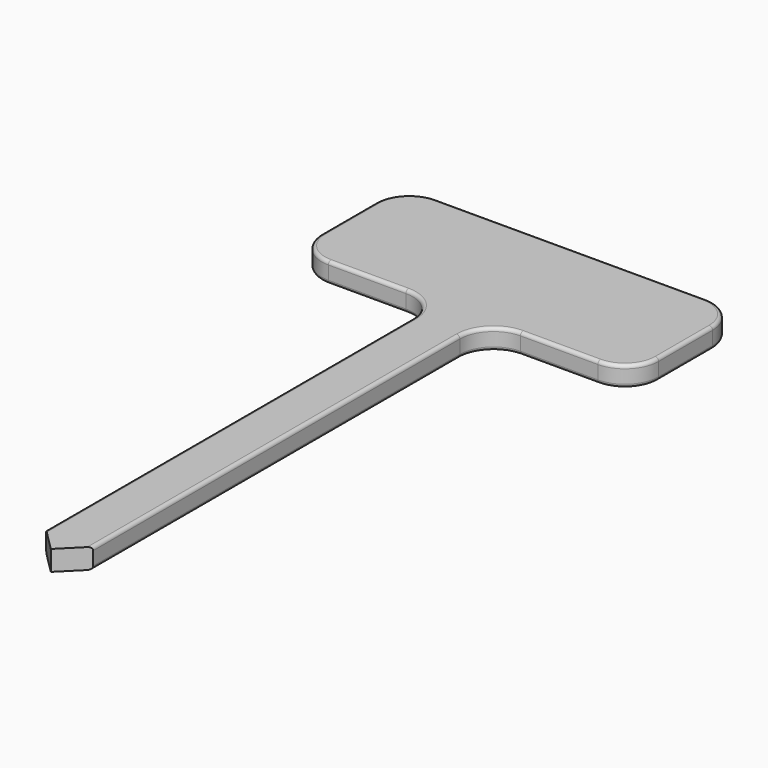
from build123d import *

# Parameters (mm, degrees)
F0_W        = 7
F0_H        = 80
F1_DEPTH    = 3
F2_R        = 5
F3_T1_DEPTH = 39.0035618315
F4_R        = 0.5


# Not quite as in the source:
# - a fillet or chamfer that OpenCascade refuses, or shapes differently, is made with other operations: its cross-section is extruded or revolved along the edge and cut away or added


with BuildPart() as f1:
    # F0 (on Top) → F1 (new body)
    with BuildSketch(Plane.XY):
        Polygon((-25, 73.9269424736), (-25, 53.9269424736), (-3.5, 53.9269424736), (3.5, 53.9269424736), (25, 53.9269424736), (25, 73.9269424736), align=None)
        with Locations((0, 13.9269424736)):
            Rectangle(F0_W, F0_H)
    extrude(amount=F1_DEPTH)

    # F2
    f2_edges = [f1.edges().sort_by_distance(p)[0] for p in [
        (-25, 73.926942, 1.5),
        (25, 73.926942, 1.5),
        (25, 53.926942, 1.5),
        (3.5, 53.926942, 1.5),
        (-3.5, 53.926942, 1.5),
        (-25, 53.926942, 1.5),
    ]]
    fillet(f2_edges, radius=F2_R)

    # F3: chamfer of 7 on 2 edges, made by hand

    # F3_s2 → F3_t1 (cut)
    with BuildSketch(Plane.XY.offset(-18.0017809158)):
        Polygon((-3.5, -19.0730575264), (3.5, -26.0730575264), (-3.5, -26.0730575264), align=None)
        Polygon((-3.5, -26.0730575264), (3.5, -19.0730575264), (3.5, -26.0730575264), align=None)
    extrude(amount=F3_T1_DEPTH, mode=Mode.SUBTRACT)

    # F4
    f4_edges = [f1.edges().sort_by_distance(p)[0] for p in [
        (-3.5, 14.926942, 3),
        (-3.5, 14.926942, 0),
    ]]
    fillet(f4_edges, radius=F4_R)


solid = f1.part
